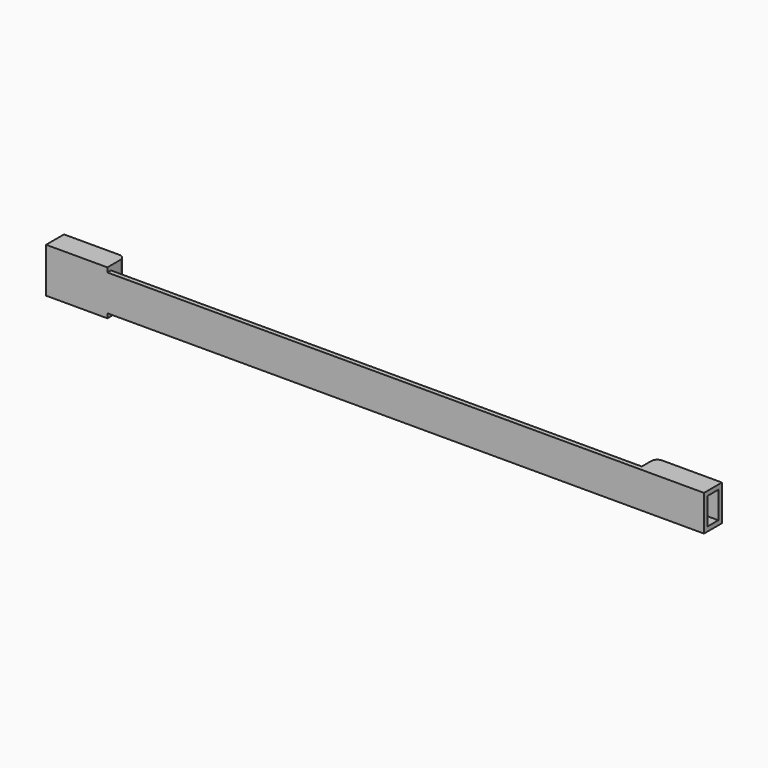
from build123d import *

# Parameters (mm, degrees)
F3_W          = 7.5
F3_H          = 12
F5_DEPTH      = 22
F4_W          = 7.5
F4_H          = 15
F6_DEPTH      = 20.5
F0_W          = 200
F0_H          = 12
F7_DEPTH      = 1.5
F8_W          = 4.5
F8_H          = 9
F9_DEPTH      = 20
F10_W         = 4.5
F10_H         = 12
F11_DEPTH     = 19
F12_TEXT_SIZE = 9.3315983476
F13_DEPTH     = 1
F14_R         = 2
F14_2_R       = 2
F16_R         = 1
F17_DEPTH     = 4
F18_R         = 1
F19_DEPTH     = 4
F20_R         = 1
F21_R         = 1
F22_TEXT_SIZE = 11.1111111111
F23_DEPTH     = 0.6


# Not quite as in the source:
# - a feature names something its author has since deleted; it is built from what else it names
# - Text() gives the source's letters only with a copy of the font that has no kerning and outlines rounded to 1/6400 em; it was checked with that copy


with BuildPart() as f5:
    # F3 (on offset) → F5 (new body)
    with BuildSketch(Plane.YZ.offset(110)):
        with Locations((3.75, 6)):
            Rectangle(F3_W, F3_H)
    extrude(amount=-F5_DEPTH)

    # F8 (on offset) → F9 (cut)
    with BuildSketch(Plane.YZ.offset(110)):
        with Locations((3.75, 6)):
            Rectangle(F8_W, F8_H)
    extrude(amount=-F9_DEPTH, mode=Mode.SUBTRACT)

    # F14#2
    f14_2_edges = [f5.edges().sort_by_distance(p)[0] for p in [
        (88, 7.5, 6),
    ]]
    fillet(f14_2_edges, radius=F14_2_R)


with BuildPart() as f6:
    # F4 (on offset) → F6 (new body)
    with BuildSketch(Plane.YZ.offset(-110)):
        with Locations((3.75, 6)):
            Rectangle(F4_W, F4_H)
    extrude(amount=F6_DEPTH)

    # F10 (on offset) → F11 (cut)
    with BuildSketch(Plane.YZ.offset(-110)):
        with Locations((3.75, 6)):
            Rectangle(F10_W, F10_H)
    extrude(amount=F11_DEPTH, mode=Mode.SUBTRACT)

    # F14
    f14_edges = [f6.edges().sort_by_distance(p)[0] for p in [
        (-89.5, 7.5, 6),
    ]]
    fillet(f14_edges, radius=F14_R)


with BuildPart() as f7:
    # F0 (on Front) → F7 (new body)
    with BuildSketch(Plane.XZ):
        with Locations((0, 6)):
            Rectangle(F0_W, F0_H)
    extrude(amount=-F7_DEPTH)

    # F12 (on face) → F13 (join)
    with BuildSketch(Plane(origin=(0, 1.5, 0), x_dir=(-1, 0, 0), z_dir=(0, 1, 0))):
        with Locations((-23.051964043, 2.9419420753)):
            Text('IES de Teis', F12_TEXT_SIZE, font='Open Sans', text_align=(TextAlign.LEFT, TextAlign.BOTTOM))
    extrude(amount=F13_DEPTH)


with BuildPart() as f5_1:
    add(f5.part)

    # F15: union F6, F7
    add(f6.part)
    add(f7.part)

    # F16 (on face) → F17 (join)
    with BuildSketch(Plane(origin=(0, 0, 0), x_dir=(1, 0, 0), z_dir=(0, 0, -1))):
        with Locations((93, -3.75)):
            Circle(F16_R)
    extrude(amount=-F17_DEPTH)

    # F18 (on face) → F19 (join)
    with BuildSketch(Plane.XY.offset(12)):
        with Locations((93, 3.75)):
            Circle(F18_R)
    extrude(amount=-F19_DEPTH)

    # F20
    f20_edges = [f5_1.edges().sort_by_distance(p)[0] for p in [
        (90, 6, 6),
    ]]
    fillet(f20_edges, radius=F20_R)

    # F21
    f21_edges = [f5_1.edges().sort_by_distance(p)[0] for p in [
        (-91, 6, 6),
    ]]
    fillet(f21_edges, radius=F21_R)

    # F22 (on face) → F23 (join)
    with BuildSketch(Plane(origin=(0, 7.5, 0), x_dir=(-1, 0, 0), z_dir=(0, 1, 0))):
        with Locations((91.8802083333, 2)):
            Text('SFS', F22_TEXT_SIZE, font='Open Sans', text_align=(TextAlign.LEFT, TextAlign.BOTTOM))
    extrude(amount=F23_DEPTH)


solid = f5_1.part
